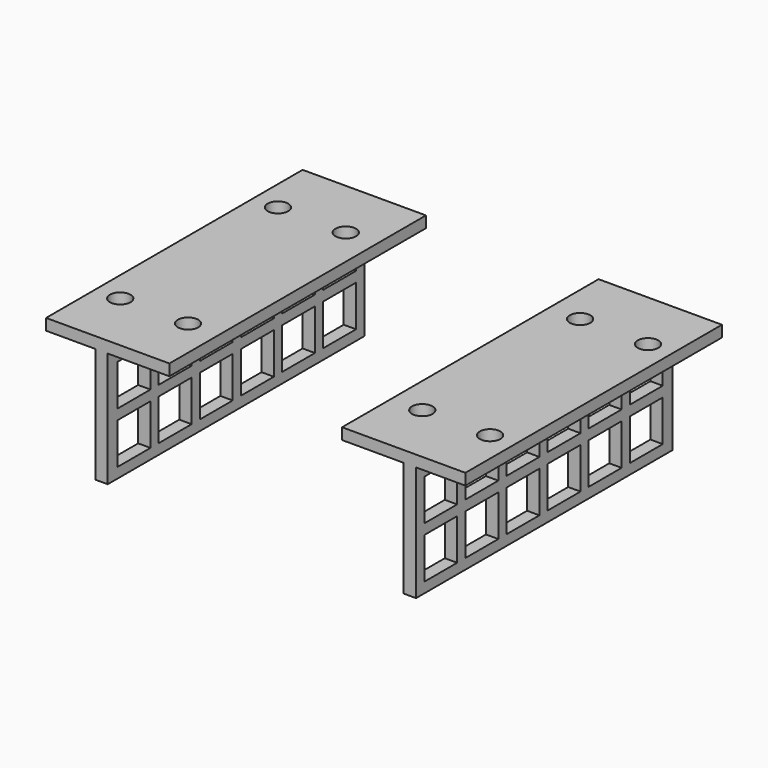
from build123d import *

# Parameters (mm, degrees)
F1_DEPTH = 39
F2_R     = 2.5
F3_DEPTH = 2.748386896
F4_W     = 10
F4_H     = 10
F5_DEPTH = 89.9998985683
F6_W     = 10
F6_H     = 10
F7_DEPTH = 89.9998985683


with BuildPart() as f1:
    # F0 (on Front) → F1 (new body, symmetric)
    with BuildSketch(Plane.XZ):
        Polygon((33.0240737289, -9.6249261405), (36.0251751605, -9.6249261405), (36.0251751605, 18.3750738595), (48.0240737289, 18.3750738595), (48.0240737289, 21.1234607555), (33.0240737289, 21.1234607555), (18.0240737289, 21.1234607555), (18.0240737289, 18.3750738595), (33.0240737289, 18.3750738595), align=None)
    extrude(amount=F1_DEPTH, both=True)


with BuildPart() as f1b:
    # F0 (on Front) → F1, piece 2 (new body, symmetric)
    with BuildSketch(Plane.XZ):
        Polygon((-53.9737234078, 21.1234607555), (-53.9737234078, 18.3750738595), (-41.9748248395, 18.3750738595), (-41.9748248395, -9.6249261405), (-38.9737234078, -9.6249261405), (-38.9737234078, 18.3750738595), (-23.9737234078, 18.3750738595), (-23.9737234078, 21.1234607555), (-38.9737234078, 21.1234607555), align=None)
    extrude(amount=F1_DEPTH, both=True)


with BuildPart() as f3_tool:
    # F2 (on face) → F3 (new body, through all)
    with BuildSketch(Plane.XY.offset(21.1234607555)):
        with Locations((42.0310314783, -23.9974405952)):
            Circle(F2_R)
        with Locations((42.051529395, 24)):
            Circle(F2_R)
        with Locations((-47.9742741236, 24)):
            Circle(F2_R)
        with Locations((-47.9742741236, -23.959002686)):
            Circle(F2_R)
        with Locations((25.5240737289, -23.9903910892)):
            Circle(F2_R)
        with Locations((25.5240737289, 24)):
            Circle(F2_R)
        with Locations((-31.4737234078, -23.9660494558)):
            Circle(F2_R)
        with Locations((-31.4737234078, 24)):
            Circle(F2_R)
    extrude(amount=-F3_DEPTH)


with BuildPart() as f1_1:
    add(f1.part)

    # F3: cut by f3_tool
    add(f3_tool.part, mode=Mode.SUBTRACT)

    # F4 (on face) → F5 (cut, through all)
    with BuildSketch(Plane.YZ.offset(36.0251751605)):
        with Locations((-31.5, -2.1249261405)):
            Rectangle(F4_W, F4_H)
        with Locations((-31.5, 10.3750738595)):
            Rectangle(F4_W, F4_H)
        with Locations((-19, -2.1249261405)):
            Rectangle(F4_W, F4_H)
        with Locations((-19, 10.3750738595)):
            Rectangle(F4_W, F4_H)
        with Locations((-6.5, -2.1249261405)):
            Rectangle(F4_W, F4_H)
        with Locations((-6.5, 10.3750738595)):
            Rectangle(F4_W, F4_H)
        with Locations((6, -2.1249261405)):
            Rectangle(F4_W, F4_H)
        with Locations((6, 10.3750738595)):
            Rectangle(F4_W, F4_H)
        with Locations((18.5, -2.1249261405)):
            Rectangle(F4_W, F4_H)
        with Locations((18.5, 10.3750738595)):
            Rectangle(F4_W, F4_H)
        with Locations((31, -2.1249261405)):
            Rectangle(F4_W, F4_H)
        with Locations((31, 10.3750738595)):
            Rectangle(F4_W, F4_H)
    extrude(amount=-F5_DEPTH, mode=Mode.SUBTRACT)


with BuildPart() as f1b_1:
    add(f1b.part)

    # F3: cut by f3_tool
    add(f3_tool.part, mode=Mode.SUBTRACT)

    # F6 (on face) → F7 (cut, through all)
    with BuildSketch(Plane(origin=(-41.9748248395, 0, 0), x_dir=(0, -1, 0), z_dir=(-1, 0, 0))):
        with Locations((-31.5, -2.1249261405)):
            Rectangle(F6_W, F6_H)
        with Locations((-31.5, 10.3750738595)):
            Rectangle(F6_W, F6_H)
        with Locations((-19, -2.1249261405)):
            Rectangle(F6_W, F6_H)
        with Locations((-19, 10.3750738595)):
            Rectangle(F6_W, F6_H)
        with Locations((-6.5, -2.1249261405)):
            Rectangle(F6_W, F6_H)
        with Locations((-6.5, 10.3750738595)):
            Rectangle(F6_W, F6_H)
        with Locations((6, -2.1249261405)):
            Rectangle(F6_W, F6_H)
        with Locations((6, 10.3750738595)):
            Rectangle(F6_W, F6_H)
        with Locations((18.5, -2.1249261405)):
            Rectangle(F6_W, F6_H)
        with Locations((18.5, 10.3750738595)):
            Rectangle(F6_W, F6_H)
        with Locations((31, -2.1249261405)):
            Rectangle(F6_W, F6_H)
        with Locations((31, 10.3750738595)):
            Rectangle(F6_W, F6_H)
    extrude(amount=-F7_DEPTH, mode=Mode.SUBTRACT)


solid = Compound([f1_1.part, f1b_1.part])
